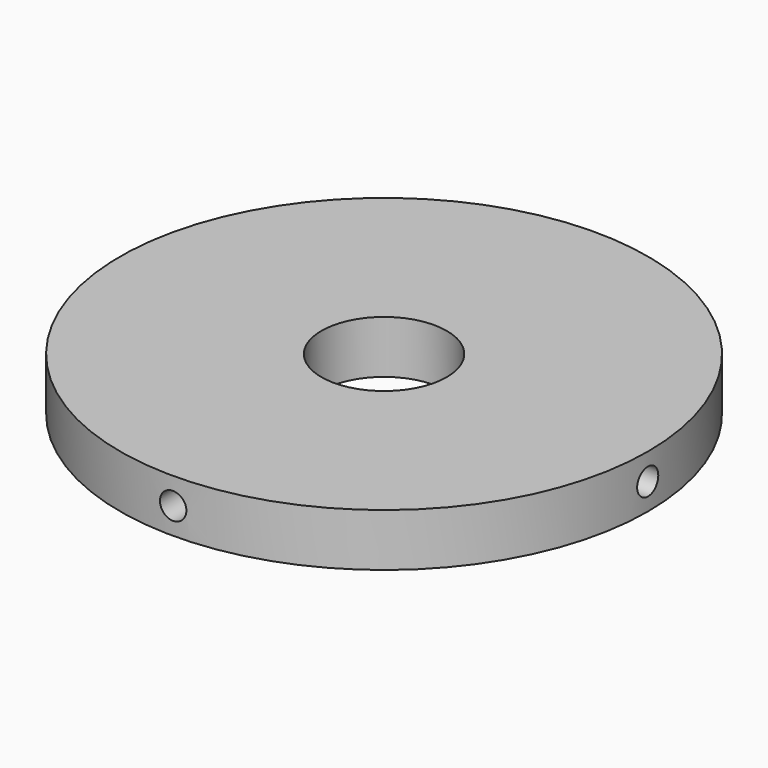
from build123d import *

# Parameters (mm, degrees)
F0_R            = 40
F1_DEPTH        = 8
F2_R            = 9.5
F3_DEPTH        = 8.001
F6_R            = 2
F7_DEPTH        = 15
F7_COPIES_COUNT = 4


# Not quite as in the source:
# - a pattern or mirror of a feature is missing from the dataset's text; its kind, count and spacing are read off the source's solid


with BuildPart() as f1:
    # F0 (on Top) → F1 (new body)
    with BuildSketch(Plane.XY):
        Circle(F0_R)
    extrude(amount=F1_DEPTH)

    # F2 (on face) → F3 (cut, through all)
    with BuildSketch(Plane.XY.offset(8)):
        Circle(F2_R)
    extrude(amount=-F3_DEPTH, mode=Mode.SUBTRACT)

    # F6 (on offset) → F7 (cut)
    with BuildSketch(Plane.XZ.offset(40.792)):
        with Locations((0, 4)):
            Circle(F6_R)
    f7 = extrude(amount=-F7_DEPTH, mode=Mode.SUBTRACT)

    # F7_copies: F7 ×4 about axis
    f7_copies_axis = Axis((0, 0, 0), (0, 0, 1))
    for i in range(1, F7_COPIES_COUNT):
        add(f7.rotate(f7_copies_axis, i * 360 / F7_COPIES_COUNT), mode=Mode.SUBTRACT)


solid = f1.part
